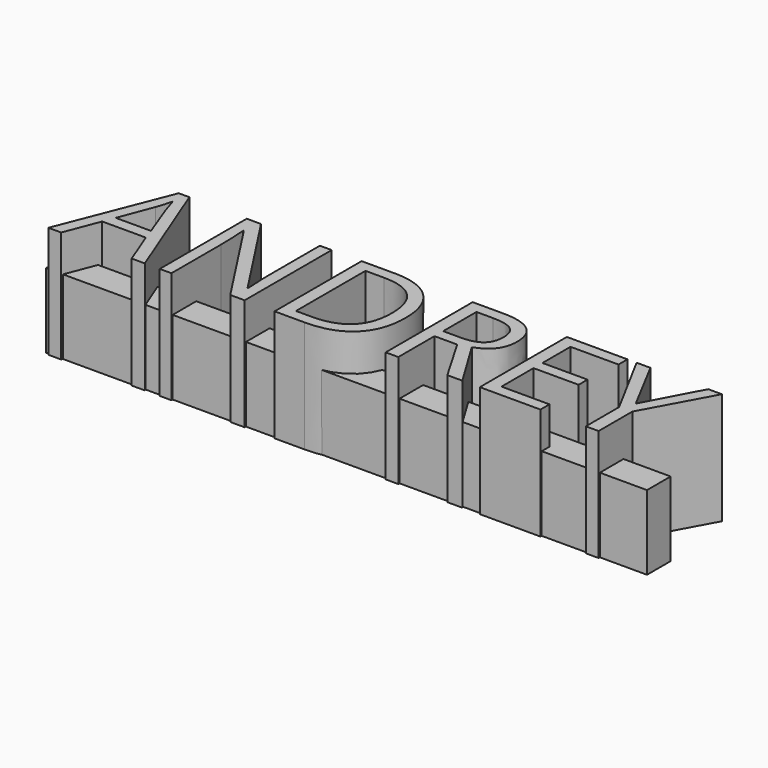
from build123d import *

# Parameters (mm, degrees)
F0_TEXT_SIZE = 20.4350429056
F2_DEPTH     = 15
F1_W         = 80.6041359901
F1_H         = 3.9608906955
F3_DEPTH     = 10


# Not quite as in the source:
# - Text() gives the source's letters only with a copy of the font that has no kerning and outlines rounded to 1/6400 em; it was checked with that copy


with BuildPart() as f2:
    # F0 (on Top) → F2 (new body)
    with BuildSketch(Plane.XY):
        with Locations((-48.4460139528, 28.7087488841)):
            Text('ANDREY', F0_TEXT_SIZE, font='Open Sans', text_align=(TextAlign.LEFT, TextAlign.BOTTOM))
    extrude(amount=F2_DEPTH)


with BuildPart() as f3:
    # F1 (on Top) → F3 (new body)
    with BuildSketch(Plane.XY):
        with Locations((-8.6149387062, 30.8949509636)):
            Rectangle(F1_W, F1_H)
    extrude(amount=F3_DEPTH)


solid = Compound([f2.part, f3.part])
